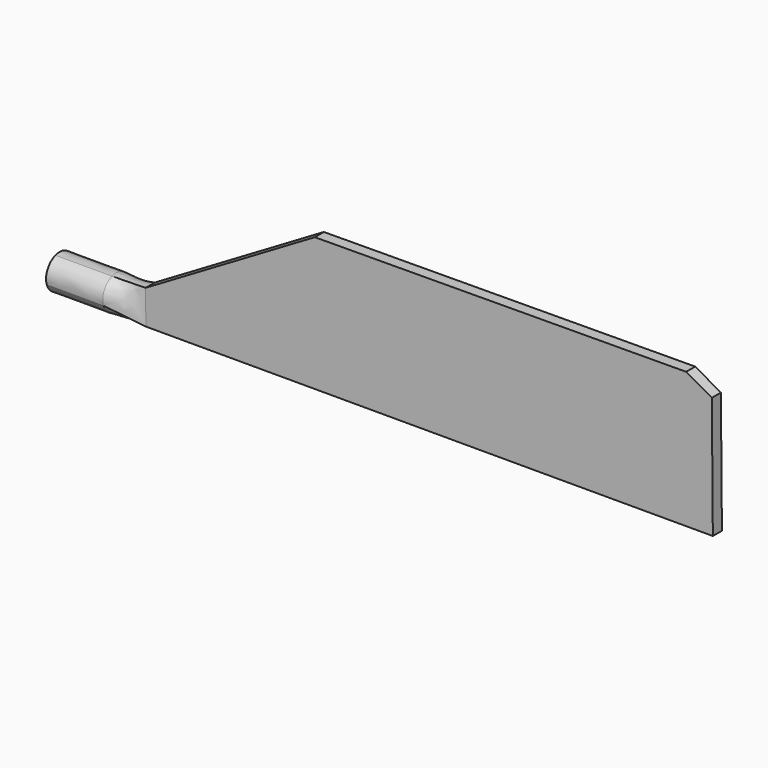
from build123d import *

# Parameters (mm, degrees)
F1_DEPTH  = 0.5
F1_FACE_W = 1
F1_FACE_H = 3
F6_DEPTH  = 5
F8_DEPTH  = 25


# Not quite as in the source:
# - the arcs of a loft's sections are written as splines that run evenly, so that the points pair up as in the source's solid


with BuildPart() as f1:
    # F0 (on Front) → F1 (new body, symmetric)
    with BuildSketch(Plane.XZ):
        Polygon((-0.0253911159, 2.9998925466), (0, 0), (50, 0), (49.8984355364, 11.9995701865), (14.899088368, 11.7857997863), align=None)
    extrude(amount=F1_DEPTH, both=True)

    # F1_face (on face) → F4 section 0
    with BuildSketch(Plane(origin=(-0.0126955579, 0, 1.4999462733), x_dir=(0, -1, 0), z_dir=(-0.9999641822, 0, -0.0084637053))):
        Rectangle(F1_FACE_W, F1_FACE_H)
    # F3 (on offset) → F4 section 1
    with BuildSketch(Plane.YZ.offset(-3)):
        with BuildLine():
            add(Edge.make_bspline(
                [(-0.4743722327, 2.9230147522), (-0.6606444281, 2.8609195721), (-0.834496694, 2.7618115588), (-1.1311572384, 2.5045080607), (-1.2538487938, 2.3464138139), (-1.4294616132, 1.995169303), (-1.482313781, 1.8021572386), (-1.5101434154, 1.4104455076), (-1.4851099322, 1.2118999628), (-1.4230147522, 1.0256277673)],
                knots=[0, 0, 0, 0, 0.25, 0.25, 0.5, 0.5, 0.75, 0.75, 1, 1, 1, 1], degree=3))
            add(Edge.make_bspline(
                [(-1.4230147522, 1.0256277673), (-1.3609195721, 0.8393555719), (-1.2618115588, 0.665503306), (-1.0045080607, 0.3688427616), (-0.8464138139, 0.2461512062), (-0.495169303, 0.0705383868), (-0.3021572386, 0.017686219), (0.0895544924, -0.0101434154), (0.2881000372, 0.0148900678), (0.4743722327, 0.0769852478)],
                knots=[0, 0, 0, 0, 0.25, 0.25, 0.5, 0.5, 0.75, 0.75, 1, 1, 1, 1], degree=3))
            add(Edge.make_bspline(
                [(0.4743722327, 0.0769852478), (0.6606444281, 0.1390804279), (0.834496694, 0.2381884412), (1.1311572384, 0.4954919393), (1.2538487938, 0.6535861861), (1.4294616132, 1.004830697), (1.482313781, 1.1978427614), (1.5101434154, 1.5895544924), (1.4851099322, 1.7881000372), (1.4230147522, 1.9743722327)],
                knots=[0, 0, 0, 0, 0.25, 0.25, 0.5, 0.5, 0.75, 0.75, 1, 1, 1, 1], degree=3))
            add(Edge.make_bspline(
                [(1.4230147522, 1.9743722327), (1.3609195721, 2.1606444281), (1.2618115588, 2.334496694), (1.0045080607, 2.6311572384), (0.8464138139, 2.7538487938), (0.495169303, 2.9294616132), (0.3021572386, 2.982313781), (-0.0895544924, 3.0101434154), (-0.2881000372, 2.9851099322), (-0.4743722327, 2.9230147522)],
                knots=[0, 0, 0, 0, 0.25, 0.25, 0.5, 0.5, 0.75, 0.75, 1, 1, 1, 1], degree=3))
        make_face()
    loft(ruled=True)

    # F5 (on face) → F6 (join)
    with BuildSketch(Plane(origin=(-3, 0, 0), x_dir=(0, -1, 0), z_dir=(-1, 0, 0))):
        with BuildLine():
            add(Edge.make_bspline(
                [(0.2236067977, 0.9472135955), (0.2049485822, 0.9590404276), (0.165567887, 0.9783654777), (0.1016629971, 0.9971413164), (0.0354857267, 0.9971906029), (-0.0298581595, 1.006417373), (-0.0962378171, 0.9979647462), (-0.1574135127, 0.9730184068), (-0.2213803356, 0.9564199077), (-0.2794920021, 0.9232440711), (-0.3264257064, 0.8766967879), (-0.3795448144, 0.8369923373), (-0.419371865, 0.7835849556), (-0.4393276132, 0.744366395), (-0.4472135955, 0.7236067977)],
                knots=[0, 0, 0, 0, 0.0661130278, 0.1311431351, 0.1976238463, 0.263561262, 0.3285913694, 0.3952621183, 0.461199534, 0.5262296414, 0.5929003903, 0.6590289395, 0.7240590469, 0.7905532518, 0.7905532518, 0.7905532518, 0.7905532518], degree=3))
            add(Edge.make_bspline(
                [(-0.4472135955, 0.7236067977), (-0.4590404276, 0.7049485822), (-0.4783654777, 0.665567887), (-0.4971413164, 0.6016629971), (-0.4971906029, 0.5354857267), (-0.506417373, 0.4701418405), (-0.4979647462, 0.4037621829), (-0.4730184068, 0.3425864873), (-0.4564199077, 0.2786196644), (-0.4232440711, 0.2205079979), (-0.3766967879, 0.1735742936), (-0.3369923373, 0.1204551856), (-0.2835849556, 0.080628135), (-0.244366395, 0.0606723868), (-0.2236067977, 0.0527864045)],
                knots=[0, 0, 0, 0, 0.0661130278, 0.1311431351, 0.1976238463, 0.263561262, 0.3285913694, 0.3952621183, 0.461199534, 0.5262296414, 0.5929003903, 0.6590289395, 0.7240590469, 0.7905532518, 0.7905532518, 0.7905532518, 0.7905532518], degree=3))
            add(Edge.make_bspline(
                [(-0.2236067977, 0.0527864045), (-0.2049485822, 0.0409595724), (-0.165567887, 0.0216345223), (-0.1016629971, 0.0028586836), (-0.0533041533, 0.0028226676), (-0.0269411852, 0.0005980705), (-0.0226951286, 0.0002149422)],
                knots=[0, 0, 0, 0, 0.0661130278, 0.1311431351, 0.1976238463, 0.2103977386, 0.2103977386, 0.2103977386, 0.2103977386], degree=3))
            add(Edge.make_bspline(
                [(0.0857219406, 0.0024530962), (0.0496252148, 0.0003925316), (0.0134550487, -0.000349593), (-0.0226951286, 0.0002149422)],
                knots=[0.7587522631, 0.7587522631, 0.7587522631, 0.7587522631, 0.8047879331, 0.8047879331, 0.8047879331, 0.8047879331], degree=3))
            add(Edge.make_bspline(
                [(0.0857219406, 0.0024530962), (0.0887772594, 0.0031276832), (0.1134683814, 0.0090615655), (0.1574135127, 0.0269815932), (0.2213803356, 0.0435800923), (0.2794920021, 0.0767559289), (0.3264257064, 0.1233032121), (0.3795448144, 0.1630076627), (0.419371865, 0.2164150444), (0.4393276132, 0.255633605), (0.4472135955, 0.2763932023)],
                knots=[0.3192274693, 0.3192274693, 0.3192274693, 0.3192274693, 0.3285913694, 0.3952621183, 0.461199534, 0.5262296414, 0.5929003903, 0.6590289395, 0.7240590469, 0.7905532518, 0.7905532518, 0.7905532518, 0.7905532518], degree=3))
            add(Edge.make_bspline(
                [(0.4472135955, 0.2763932023), (0.4590404276, 0.2950514178), (0.4783654777, 0.334432113), (0.4971413164, 0.3983370029), (0.4971906029, 0.4645142733), (0.506417373, 0.5298581595), (0.4979647462, 0.5962378171), (0.4730184068, 0.6574135127), (0.4564199077, 0.7213803356), (0.4232440711, 0.7794920021), (0.3766967879, 0.8264257064), (0.3369923373, 0.8795448144), (0.2835849556, 0.919371865), (0.244366395, 0.9393276132), (0.2236067977, 0.9472135955)],
                knots=[0, 0, 0, 0, 0.0661130278, 0.1311431351, 0.1976238463, 0.263561262, 0.3285913694, 0.3952621183, 0.461199534, 0.5262296414, 0.5929003903, 0.6590289395, 0.7240590469, 0.7905532518, 0.7905532518, 0.7905532518, 0.7905532518], degree=3))
        make_face()
        with BuildLine():
            add(Edge.make_bspline(
                [(-0.4472135955, 0.7236067977), (-0.4590404276, 0.7049485822), (-0.4783654777, 0.665567887), (-0.4971413164, 0.6016629971), (-0.4971906029, 0.5354857267), (-0.506417373, 0.4701418405), (-0.4979647462, 0.4037621829), (-0.4730184068, 0.3425864873), (-0.4564199077, 0.2786196644), (-0.4232440711, 0.2205079979), (-0.3766967879, 0.1735742936), (-0.3369923373, 0.1204551856), (-0.2835849556, 0.080628135), (-0.244366395, 0.0606723868), (-0.2236067977, 0.0527864045)],
                knots=[0, 0, 0, 0, 0.0661130278, 0.1311431351, 0.1976238463, 0.263561262, 0.3285913694, 0.3952621183, 0.461199534, 0.5262296414, 0.5929003903, 0.6590289395, 0.7240590469, 0.7905532518, 0.7905532518, 0.7905532518, 0.7905532518], degree=3))
            add(Edge.make_bspline(
                [(0.2236067977, 0.9472135955), (0.2049485822, 0.9590404276), (0.165567887, 0.9783654777), (0.1016629971, 0.9971413164), (0.0354857267, 0.9971906029), (-0.0298581595, 1.006417373), (-0.0962378171, 0.9979647462), (-0.1574135127, 0.9730184068), (-0.2213803356, 0.9564199077), (-0.2794920021, 0.9232440711), (-0.3264257064, 0.8766967879), (-0.3795448144, 0.8369923373), (-0.419371865, 0.7835849556), (-0.4393276132, 0.744366395), (-0.4472135955, 0.7236067977)],
                knots=[0, 0, 0, 0, 0.0661130278, 0.1311431351, 0.1976238463, 0.263561262, 0.3285913694, 0.3952621183, 0.461199534, 0.5262296414, 0.5929003903, 0.6590289395, 0.7240590469, 0.7905532518, 0.7905532518, 0.7905532518, 0.7905532518], degree=3))
            add(Edge.make_bspline(
                [(0.4472135955, 0.2763932023), (0.4590404276, 0.2950514178), (0.4783654777, 0.334432113), (0.4971413164, 0.3983370029), (0.4971906029, 0.4645142733), (0.506417373, 0.5298581595), (0.4979647462, 0.5962378171), (0.4730184068, 0.6574135127), (0.4564199077, 0.7213803356), (0.4232440711, 0.7794920021), (0.3766967879, 0.8264257064), (0.3369923373, 0.8795448144), (0.2835849556, 0.919371865), (0.244366395, 0.9393276132), (0.2236067977, 0.9472135955)],
                knots=[0, 0, 0, 0, 0.0661130278, 0.1311431351, 0.1976238463, 0.263561262, 0.3285913694, 0.3952621183, 0.461199534, 0.5262296414, 0.5929003903, 0.6590289395, 0.7240590469, 0.7905532518, 0.7905532518, 0.7905532518, 0.7905532518], degree=3))
            add(Edge.make_bspline(
                [(0.0857219406, 0.0024530962), (0.0887772594, 0.0031276832), (0.1134683814, 0.0090615655), (0.1574135127, 0.0269815932), (0.2213803356, 0.0435800923), (0.2794920021, 0.0767559289), (0.3264257064, 0.1233032121), (0.3795448144, 0.1630076627), (0.419371865, 0.2164150444), (0.4393276132, 0.255633605), (0.4472135955, 0.2763932023)],
                knots=[0.3192274693, 0.3192274693, 0.3192274693, 0.3192274693, 0.3285913694, 0.3952621183, 0.461199534, 0.5262296414, 0.5929003903, 0.6590289395, 0.7240590469, 0.7905532518, 0.7905532518, 0.7905532518, 0.7905532518], degree=3))
            add(Edge.make_bspline(
                [(1.4230147522, 1.0256277673), (1.3609195721, 0.8393555719), (1.2618115588, 0.665503306), (1.0045080607, 0.3688427616), (0.8464138139, 0.2461512062), (0.495169303, 0.0705383868), (0.3021572386, 0.017686219), (0.0994446448, 0.0032842572), (0.09258462, 0.002844849), (0.0857219406, 0.0024530962)],
                knots=[0, 0, 0, 0, 0.25, 0.25, 0.5, 0.5, 0.75, 0.75, 0.7587522631, 0.7587522631, 0.7587522631, 0.7587522631], degree=3))
            add(Edge.make_bspline(
                [(0.4743722327, 2.9230147522), (0.6606444281, 2.8609195721), (0.834496694, 2.7618115588), (1.1311572384, 2.5045080607), (1.2538487938, 2.3464138139), (1.4294616132, 1.995169303), (1.482313781, 1.8021572386), (1.5101434154, 1.4104455076), (1.4851099322, 1.2118999628), (1.4230147522, 1.0256277673)],
                knots=[0, 0, 0, 0, 0.25, 0.25, 0.5, 0.5, 0.75, 0.75, 1, 1, 1, 1], degree=3))
            add(Edge.make_bspline(
                [(-1.4230147522, 1.9743722327), (-1.3609195721, 2.1606444281), (-1.2618115588, 2.334496694), (-1.0045080607, 2.6311572384), (-0.8464138139, 2.7538487938), (-0.495169303, 2.9294616132), (-0.3021572386, 2.982313781), (0.0895544924, 3.0101434154), (0.2881000372, 2.9851099322), (0.4743722327, 2.9230147522)],
                knots=[0, 0, 0, 0, 0.25, 0.25, 0.5, 0.5, 0.75, 0.75, 1, 1, 1, 1], degree=3))
            add(Edge.make_bspline(
                [(-0.4743722327, 0.0769852478), (-0.6606444281, 0.1390804279), (-0.834496694, 0.2381884412), (-1.1311572384, 0.4954919393), (-1.2538487938, 0.6535861861), (-1.4294616132, 1.004830697), (-1.482313781, 1.1978427614), (-1.5101434154, 1.5895544924), (-1.4851099322, 1.7881000372), (-1.4230147522, 1.9743722327)],
                knots=[0, 0, 0, 0, 0.25, 0.25, 0.5, 0.5, 0.75, 0.75, 1, 1, 1, 1], degree=3))
            add(Edge.make_bspline(
                [(-0.0226951286, 0.0002149422), (-0.1759882345, 0.002608827), (-0.3289219115, 0.0284983341), (-0.4743722327, 0.0769852478)],
                knots=[0.8047879331, 0.8047879331, 0.8047879331, 0.8047879331, 1, 1, 1, 1], degree=3))
            add(Edge.make_bspline(
                [(-0.2236067977, 0.0527864045), (-0.2049485822, 0.0409595724), (-0.165567887, 0.0216345223), (-0.1016629971, 0.0028586836), (-0.0533041533, 0.0028226676), (-0.0269411852, 0.0005980705), (-0.0226951286, 0.0002149422)],
                knots=[0, 0, 0, 0, 0.0661130278, 0.1311431351, 0.1976238463, 0.2103977386, 0.2103977386, 0.2103977386, 0.2103977386], degree=3))
        make_face()
    extrude(amount=F6_DEPTH)

    # F7 (on face) → F8 (cut)
    with BuildSketch(Plane.XZ.offset(0.5)):
        Polygon((49.8984355364, 11.9995701865), (47.6442072011, 11.9858017213), (49.9094060968, 10.7034277653), align=None)
    extrude(amount=-F8_DEPTH, mode=Mode.SUBTRACT)


solid = f1.part
